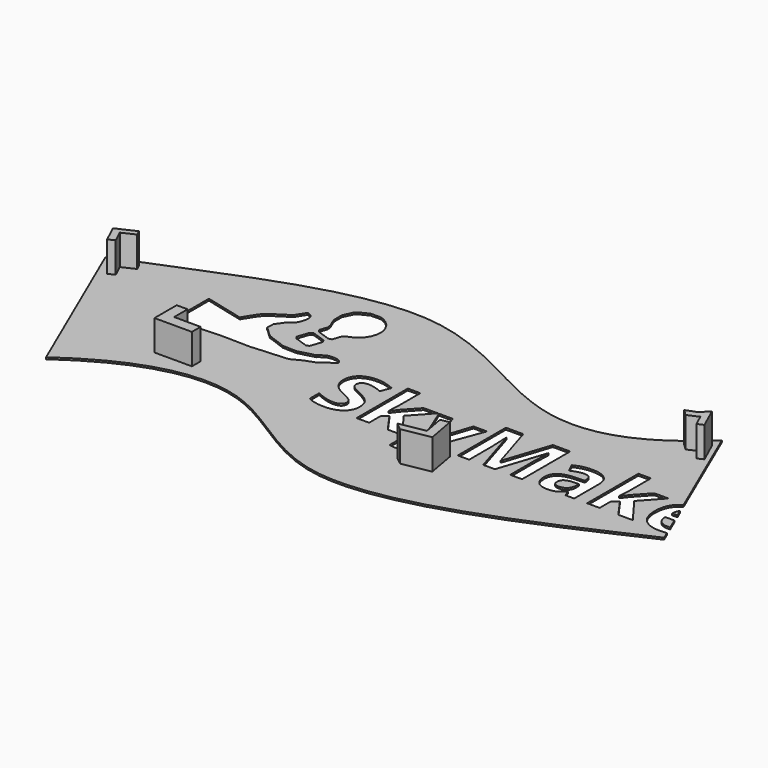
from build123d import *

# Parameters (mm, degrees)
F1_DEPTH     = 0.6
F3_DEPTH     = 10
F5_DEPTH     = 15
F6_TEXT_SIZE = 27.7777777778
F7_DEPTH     = 12.5


# Not quite as in the source:
# - Text() gives the source's letters only with a copy of the font that has no kerning and outlines rounded to 1/6400 em; it was checked with that copy


with BuildPart() as f1:
    # F0 (on Top) → F1 (new body)
    with BuildSketch(Plane.XY):
        with BuildLine():
            Line((-63.8958341201, 24.4100193448), (-41.018165648, -28.620665893))
            add(Edge.make_bspline(
                [(-41.018165648, -28.620665893), (-20.4457198492, -13.9450909045), (13.6398545362, -6.6271954206), (52.7990907234, -50.6223213151), (113.9659349305, -22.5634761348), (146.036875872, -7.8036431615)],
                knots=[0, 0, 0, 0, 0.3084506284, 0.5906321497, 1, 1, 1, 1], degree=3))
            Line((146.036875872, -7.8036431615), (123.7372105094, 43.887224559))
            add(Edge.make_bspline(
                [(123.7372105094, 43.887224559), (106.3881437267, 27.1657273507), (74.6079144736, 20.7892123266), (22.7329883038, 64.7015032543), (-35.2993587342, 35.5190691377), (-63.8958341201, 24.4100193448)],
                knots=[0, 0, 0, 0, 0.2943413391, 0.6064594547, 1, 1, 1, 1], degree=3))
        make_face()
    extrude(amount=F1_DEPTH)

    # F2 (on face) → F3 (join)
    with BuildSketch(Plane.XY.offset(0.6)):
        Polygon((-60.4699328542, 23.2431814075), (-57.7697381377, 17.4570474774), (-55.7237102674, 18.4547206708), (-57.5922723456, 22.4587839242), (-53.4110518567, 24.4100193448), (-54.2262598236, 26.1568942824), align=None)
        Polygon((123.7372105094, 39.7015176713), (120.7003518939, 37.1299013495), (117.6144108176, 35.9726771712), (119.6186456783, 34.0328778499), (123.2261297088, 35.6617031613), (124.9325480328, 31.8823679496), (126.8722265959, 32.7581577003), align=None)
        Polygon((64.6292216194, -15.9882377425), (67.2107562423, -18.0312395096), (76.4685720205, -16.3596905768), (74.7807854832, -7.011943389), (71.9288971579, -7.5268673193), (73.1779526641, -14.4447179106), align=None)
        Polygon((-20.8670608699, 0), (-20.8670608699, -2.8587111738), (-20.8670608699, -9.1591682285), (-8.523308672, -9.1591682285), (-8.523308672, -5.5589070544), (-17.2667987645, -5.5589070544), (-17.2667987645, 0), align=None)
    extrude(amount=F3_DEPTH)

    # F4 (on Top) → F5 (cut, symmetric)
    with BuildSketch(Plane.XY):
        Polygon((-15.9081370251, 19.8267707697), (-28.663339145, 23.0385759159), (-28.663339145, 8.0385759159), (-26.6870993831, 8.1767097069), (-22.051660368, 8.476034952), (-16.7063141022, 8.7676507331), (-13.540624282, 8.8981457891), (-12.5888944858, 8.8904363251), (-12.0785845512, 8.8904363251), (-10.5398038253, 8.8636300236), (-7.7232324857, 8.8098759626), (-5.0562530395, 8.7600119981), (-3.7055407982, 8.7446637991), (-3.4446214152, 8.7523025341), (-3.1452961701, 8.7638313656), (-1.1537789381, 8.9173133556), (0.8147513598, 9.0938530087), (1.1025477734, 9.1130205752), (1.3864540904, 9.1360782382), (2.7602947238, 9.2051097692), (4.3028948172, 9.2933795957), (4.6750709607, 9.3202566262), (5.1701034254, 9.3624111267), (7.1041179578, 9.4430422182), (8.6044928217, 9.6809746673), (8.8808311327, 9.7998701628), (9.0650095208, 9.8766111578), (10.0357654255, 10.4061593879), (11.2061186462, 11.0393256436), (11.4900956923, 11.1621112356), (11.8969290594, 11.3463603527), (13.4855737498, 11.9487594813), (14.5714765115, 12.3248257214), (14.7326679656, 12.3977473489), (14.8898985941, 12.4744883439), (15.7341909973, 13.0845969366), (16.8239838556, 13.9172897793), (17.1040708051, 14.1015388963), (17.3842284837, 14.2857172844), (18.873074516, 15.1682740916), (19.7325736602, 15.8897101737), (19.6981286237, 15.9932574702), (19.5983299657, 16.2734151488), (18.9843312766, 16.9909611345), (17.8753708518, 17.4475877371), (16.543826177, 17.5128706296), (15.5038972832, 17.3900143086), (15.1662369052, 17.3209827776), (14.9512913901, 17.278757548), (14.3489629905, 16.979503032), (13.4893931173, 16.4153683073), (12.8101822646, 15.8858200772), (12.5376633211, 15.6479583572), (12.107913749, 15.5750367297), (7.925281969, 14.4890632389), (7.5185193309, 14.3432907129), (6.9851517333, 14.3010654834), (4.5522853687, 14.3586389119), (2.7333469643, 14.4430186419), (2.5147235397, 14.4123222439), (2.0503167441, 14.6349064939), (-2.7500623635, 16.4000201083), (-3.2450948281, 16.5305151644), (-3.4292732162, 16.6494813889), (-5.0409048405, 18.0923535533), (-5.175219264, 18.2572936458), (-5.3018242236, 18.4146657323), (-6.8022698164, 19.7307914791), (-6.974990102, 19.8344095046), (-6.8328954854, 22.2711659657), (-4.983331412, 24.9227264839), (-4.7799854575, 25.0455120759), (-2.9957042766, 26.6110283742), (-2.845970925, 26.7952067622), (-2.661792537, 27.0984221038), (-2.2128753984, 28.0730681051), (-1.7907645613, 29.5274691009), (-1.7677068983, 30.9049876437), (-2.1169668369, 31.7721962519), (-2.3241321589, 31.9525552725), (-2.600399741, 32.194307089), (-3.6364385382, 32.6625332522), (-4.0317430738, 32.5703733291), (-4.1584187623, 32.317092681), (-5.6894900242, 29.9457605705), (-5.8698490447, 29.7269249589), (-6.1154202288, 29.4507281059), (-7.0402022655, 28.7945041872), (-8.7822582169, 27.712350064), (-10.8391290704, 26.3233026897), (-12.4737476287, 24.9764098159), (-12.9610706294, 24.4737386162), (-13.2757440734, 24.1360075091), (-15.7354167395, 20.2565203417), align=None)
        Polygon((8.0366094585, 18.6832238504), (9.3373870063, 22.4859700228), (8.8154775112, 23.383945758), (4.4524867107, 24.8727917903), (3.481730806, 24.3931075247), (2.1924113607, 20.6057802804), (2.7947397603, 19.7462104071), (7.1194661568, 18.2649323808), align=None)
        Polygon((14.283750827, 29.6464353255), (14.4870967815, 29.750053351), (14.8976787871, 30.0147921015), (15.9874009164, 31.0470115313), (17.0542068406, 32.6817008186), (17.6336190352, 34.5427937236), (17.7334176933, 36.0393492199), (17.6758442648, 36.5266722205), (17.6144514688, 37.0139952212), (17.1577541371, 38.445267825), (16.1524117379, 40.1144728779), (14.7288485981, 41.4460882817), (13.4241809538, 42.1866919304), (12.9598448872, 42.3440640169), (12.3190398965, 42.5626874414), (9.0688288883, 42.5358811399), (6.1447494266, 41.1084279036), (5.672774625, 40.6249242705), (5.1969804559, 40.1452400049), (3.8078623525, 37.2058830732), (3.8232105515, 33.9518526974), (4.0496141691, 33.3148670743), (4.1301745316, 33.0576963297), (4.2605988586, 32.7353841506), (4.9743962058, 31.2043128888), (5.2085092874, 29.6924799225), (5.1010011653, 29.3739163819), (4.3642876132, 27.1636342673), (4.9705768383, 26.3002450266), (9.1916144803, 24.8267471933), (10.2659884105, 25.1145436069), (11.0027726917, 27.3708703184), (11.1102808138, 27.6931824975), (12.3036209685, 28.6908861617), (13.9498390874, 29.4469087384), align=None)
    extrude(amount=F5_DEPTH, both=True, mode=Mode.SUBTRACT)

    # F6 (on face) → F7 (cut, symmetric)
    with BuildSketch(Plane.XY.offset(0.6)):
        with Locations((25.1131284931, -5.2085771481)):
            Text('SkyMaker', F6_TEXT_SIZE, font='Open Sans', font_style=FontStyle.BOLD, text_align=(TextAlign.LEFT, TextAlign.BOTTOM))
    extrude(amount=F7_DEPTH, both=True, mode=Mode.SUBTRACT)


solid = f1.part
